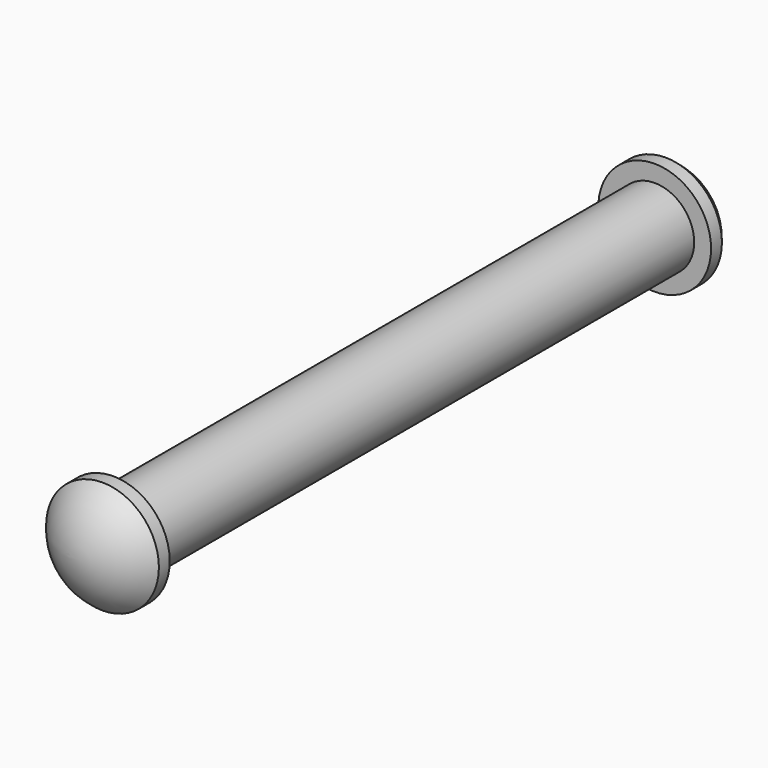
from build123d import *

# Parameters (mm, degrees)
F0_R     = 1.75
F1_DEPTH = 15
F2_R     = 2.5
F2_R_2   = 1.75
F3_DEPTH = 0.6


# Not quite as in the source:
# - a pattern or mirror of a feature is missing from the dataset's text; its kind, count and spacing are read off the source's solid


with BuildPart() as f1:
    # F0 (on Front) → F1 (new body, symmetric)
    with BuildSketch(Plane.XZ):
        Circle(F0_R)
    extrude(amount=F1_DEPTH, both=True)

    # F2 (on face) → F3 (join)
    with BuildSketch(Plane.XZ.offset(15)):
        Circle(F2_R)
        Circle(F2_R_2, mode=Mode.SUBTRACT)
        Circle(F2_R_2)
    f3 = extrude(amount=F3_DEPTH)

    # F3_copies: F3 across plane
    add(f3.mirror(Plane.ZX))

    # F4 (on Top) → F5 (revolve)
    with BuildSketch(Plane.XY):
        with BuildLine():
            Line((0, -16.9), (0, -15.6))
            Line((0, -15.6), (-2.5, -15.6))
            ThreePointArc((-2.5, -15.6), (-1.4089002804, -16.5555774622), (0, -16.9))
        make_face()
    f5 = revolve(axis=Axis((0, -16.1810277431, 0), (0, -1, 0)))

    # F5_copies: F5 across plane
    add(f5.mirror(Plane.ZX))


solid = f1.part
